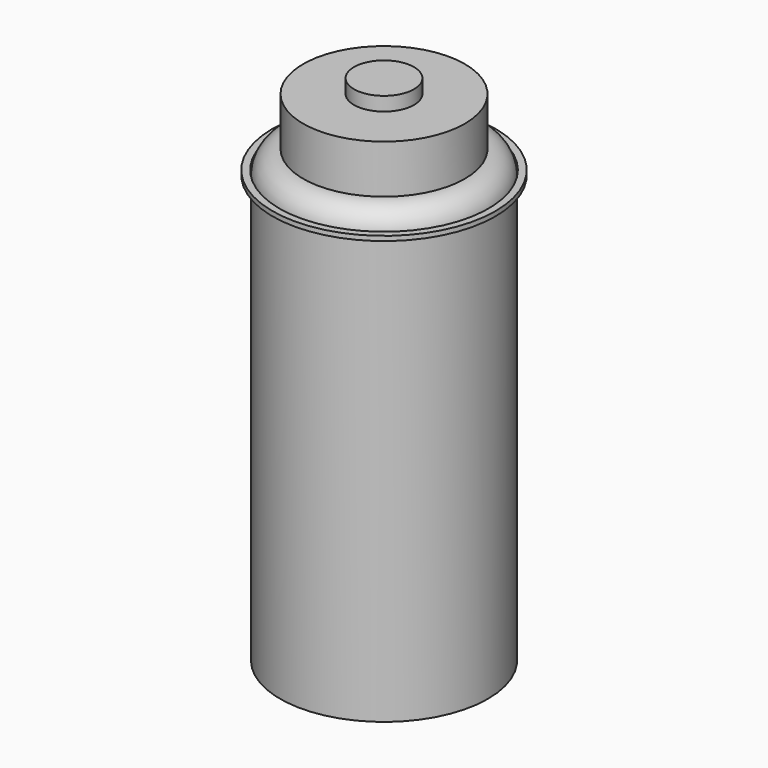
from build123d import *

# Parameters (mm, degrees)
F0_R      = 45
F1_DEPTH  = 195
F2_R      = 10
F3_R      = 35
F4_DEPTH  = 21
F5_W      = 3
F5_H      = 2
F7_R      = 13
F8_DEPTH  = 3
F9_R      = 13
F10_DEPTH = 3


with BuildPart() as f1:
    # F0 (on Top) → F1 (new body)
    with BuildSketch(Plane.XY):
        Circle(F0_R)
    extrude(amount=F1_DEPTH)

    # F2
    f2_edges = [f1.edges().sort_by_distance(p)[0] for p in [
        (-45, 0, 195),
    ]]
    fillet(f2_edges, radius=F2_R)

    # F3 (on face) → F4 (join)
    with BuildSketch(Plane.XY.offset(195)):
        Circle(F3_R)
    extrude(amount=F4_DEPTH)

    # F7 (on face) → F8 (join)
    with BuildSketch(Plane.XY.offset(216)):
        Circle(F7_R)
    extrude(amount=F8_DEPTH)

    # F9 (on face) → F10 (join)
    with BuildSketch(Plane.XY.offset(219)):
        Circle(F9_R)
    extrude(amount=F10_DEPTH)


with BuildPart() as f6:
    # F5 (on Front) → F6 (revolve)
    with BuildSketch(Plane.XZ):
        with Locations((-46.7765510678, 186)):
            Rectangle(F5_W, F5_H)
    revolve(axis=Axis((0, 0, 185), (0, 0, 1)))


solid = Compound([f1.part, f6.part])
